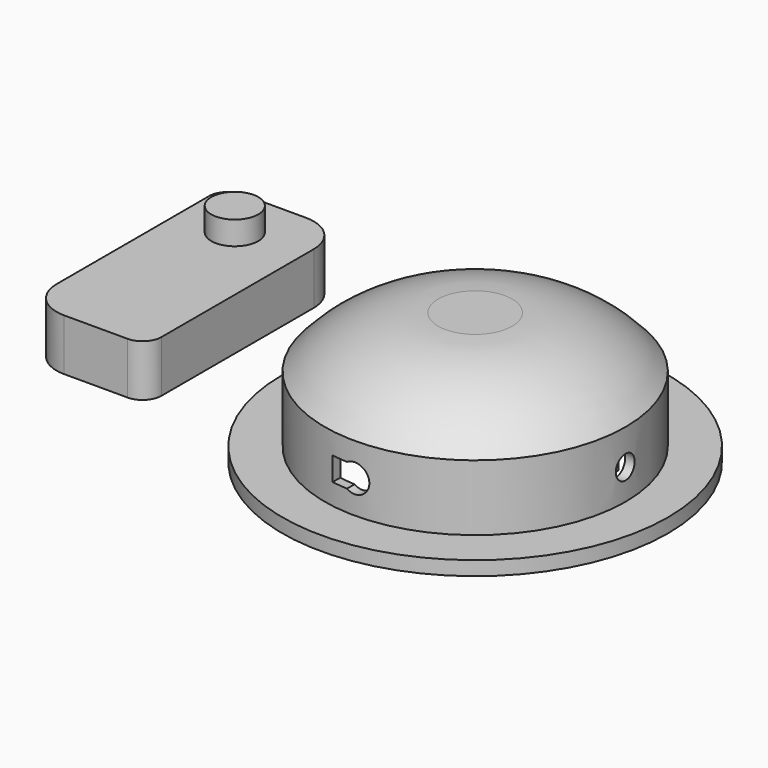
from build123d import *

# Parameters (mm, degrees)
F0_R      = 41
F1_DEPTH  = 3
F2_R      = 32
F3_DEPTH  = 14
F4_R      = 32
F5_DEPTH  = 11
F9_DEPTH  = 120.3
F11_R     = 2.5
F12_DEPTH = 58.4
F13_R     = 40.25
F13_R_2   = 39.25
F14_DEPTH = 1
F15_R     = 39.25
F15_R_2   = 38.75
F16_DEPTH = 0.5
F17_R     = 30
F18_DEPTH = 15
F20_DEPTH = 4.5
F22_DEPTH = 11
F24_DEPTH = 15
F26_DEPTH = 5
F28_DEPTH = 11
F29_R     = 5
F30_DEPTH = 5


# Not quite as in the source:
# - a fillet or chamfer that OpenCascade refuses, or shapes differently, is made with other operations: its cross-section is extruded or revolved along the edge and cut away or added


with BuildPart() as f1:
    # F0 (on Top) → F1 (new body)
    with BuildSketch(Plane.XY):
        Circle(F0_R)
    extrude(amount=F1_DEPTH)

    # F13 (on face) → F14 (cut)
    with BuildSketch(Plane(origin=(0, 0, 0), x_dir=(1, 0, 0), z_dir=(0, 0, -1))):
        Circle(F13_R)
        Circle(F13_R_2, mode=Mode.SUBTRACT)
    extrude(amount=-F14_DEPTH, mode=Mode.SUBTRACT)

    # F15 (on face) → F16 (join)
    with BuildSketch(Plane(origin=(0, 0, 0), x_dir=(1, 0, 0), z_dir=(0, 0, -1))):
        Circle(F15_R)
        Circle(F15_R_2, mode=Mode.SUBTRACT)
    extrude(amount=F16_DEPTH)


with BuildPart() as f3:
    # F2 (on face) → F3 (new body)
    with BuildSketch(Plane.XY.offset(3)):
        Circle(F2_R)
    extrude(amount=F3_DEPTH)

    # F8 (on offset) → F9 (cut)
    with BuildSketch(Plane.XZ.offset(55.4)):
        with BuildLine():
            ThreePointArc((-1.6706518419, 7.5), (1.4062977188, 7.3566179631), (2.9876605533, 10))
            ThreePointArc((2.9876605533, 10), (1.4062977188, 12.6433820369), (-1.6706518419, 12.5))
            ThreePointArc((-1.6706518419, 12.5), (-3.0123394467, 10), (-1.6706518419, 7.5))
        make_face()
        with BuildLine():
            ThreePointArc((-1.6706518419, 7.5), (-3.0123394467, 10), (-1.6706518419, 12.5))
            Line((-1.6706518419, 12.5), (-5.0123394467, 12.5))
            Line((-5.0123394467, 12.5), (-5.0123394467, 10))
            Line((-5.0123394467, 10), (-5.0123394467, 7.5))
            Line((-5.0123394467, 7.5), (-1.6706518419, 7.5))
        make_face()
    extrude(amount=-F9_DEPTH, mode=Mode.SUBTRACT)

    # F11 (on offset) → F12 (cut)
    with BuildSketch(Plane.YZ.offset(56.8)):
        with Locations((0, 9.5)):
            Circle(F11_R)
    extrude(amount=-F12_DEPTH, mode=Mode.SUBTRACT)


with BuildPart() as f5:
    # F4 (on face) → F5 (new body)
    with BuildSketch(Plane.XY.offset(17)):
        Circle(F4_R)
    extrude(amount=F5_DEPTH)

    # F6: fillet of radius 32 on 1 edges, made by hand

    # F6_s1 → F6_t2 (revolve, cut)
    with BuildSketch(Plane.XZ):
        with BuildLine():
            ThreePointArc((32, 17), (21.1211062261, 25.1204395571), (7.8546070647, 28))
            Line((7.8546070647, 28), (32, 28))
            Line((32, 28), (32, 17))
        make_face()
    revolve(axis=Axis((0, 0, 28), (0, 0, 1)), mode=Mode.SUBTRACT)


with BuildPart() as f18_tool:
    # F17 (on face) → F18 (new body)
    with BuildSketch(Plane(origin=(0, 0, 0), x_dir=(1, 0, 0), z_dir=(0, 0, -1))):
        Circle(F17_R)
    extrude(amount=-F18_DEPTH)


with BuildPart() as f1_1:
    add(f1.part)

    # F18: cut by f18_tool
    add(f18_tool.part, mode=Mode.SUBTRACT)

    # F19 (on face) → F20 (join)
    with BuildSketch(Plane(origin=(0, 0, 0), x_dir=(1, 0, 0), z_dir=(0, 0, -1))):
        Polygon((32, 5), (32, 0), (32, -5), (33, -5), (33, 5), align=None)
    extrude(amount=F20_DEPTH)

    # F25 (on face) → F26 (join)
    with BuildSketch(Plane(origin=(0, 0, 0), x_dir=(1, 0, 0), z_dir=(0, 0, -1))):
        with BuildLine():
            Line((5, 30.5941170816), (5, 31.6069612586))
            ThreePointArc((5, 31.6069612586), (0, 32), (-5, 31.6069612586))
            Line((-5, 31.6069612586), (-5, 30.5941170816))
            ThreePointArc((-5, 30.5941170816), (0, 31), (5, 30.5941170816))
        make_face()
        with BuildLine():
            ThreePointArc((-5, -31.6069612586), (0, -32), (5, -31.6069612586))
            Line((5, -31.6069612586), (5, -30.5941170816))
            ThreePointArc((5, -30.5941170816), (0, -31), (-5, -30.5941170816))
            Line((-5, -30.5941170816), (-5, -31.6069612586))
        make_face()
        with BuildLine():
            ThreePointArc((-31.8590646441, -3), (-31.5207631121, -5.5173809756), (-30.9838667697, -8))
            Line((-30.9838667697, -8), (-29.9499582637, -8))
            ThreePointArc((-29.9499582637, -8), (-30.504843096, -5.5185639156), (-30.8544972411, -3))
            Line((-30.8544972411, -3), (-31.8590646441, -3))
        make_face()
        with BuildLine():
            Line((-29.9499582637, 8), (-30.9838667697, 8))
            ThreePointArc((-30.9838667697, 8), (-31.7449502805, 4.0321373594), (-32, 0))
            Line((-32, 0), (-31, 0))
            ThreePointArc((-31, 0), (-30.7363685735, 4.0343087279), (-29.9499582637, 8))
        make_face()
        with BuildLine():
            Line((-31, 0), (-32, 0))
            ThreePointArc((-32, 0), (-31.9960925573, -0.5000610612), (-31.9843711834, -1))
            Line((-31.9843711834, -1), (-30.9838667697, -1))
            ThreePointArc((-30.9838667697, -1), (-30.99596643, -0.500065066), (-31, 0))
        make_face()
    extrude(amount=F26_DEPTH)


with BuildPart() as f3_1:
    add(f3.part)

    # F18: cut by f18_tool
    add(f18_tool.part, mode=Mode.SUBTRACT)

    # F21 (on face) → F22 (join)
    with BuildSketch(Plane(origin=(0, 0, 15), x_dir=(1, 0, 0), z_dir=(0, 0, -1))):
        with BuildLine():
            ThreePointArc((25.25, 6.125), (23.1161165235, 7.0088834765), (24, 4.875))
            ThreePointArc((24, 4.875), (24.8838834765, 5.2411165235), (25.25, 6.125))
        make_face()
        with BuildLine():
            ThreePointArc((24.75, 6.125), (24.5303300859, 5.5946699141), (24, 5.375))
            ThreePointArc((24, 5.375), (23.4696699141, 6.6553300859), (24.75, 6.125))
        make_face(mode=Mode.SUBTRACT)
        with BuildLine():
            ThreePointArc((25.25, -6.125), (24.8838834765, -5.2411165235), (24, -4.875))
            ThreePointArc((24, -4.875), (23.1161165235, -7.0088834765), (25.25, -6.125))
        make_face()
        with BuildLine():
            ThreePointArc((24.75, -6.125), (23.4696699141, -6.6553300859), (24, -5.375))
            ThreePointArc((24, -5.375), (24.5303300859, -5.5946699141), (24.75, -6.125))
        make_face(mode=Mode.SUBTRACT)
    extrude(amount=F22_DEPTH)


with BuildPart() as f24:
    # F23 (on face) → F24 (new body, through all)
    with BuildSketch(Plane(origin=(0, 0, 0), x_dir=(1, 0, 0), z_dir=(0, 0, -1))):
        with BuildLine():
            Line((19.5, 20.25), (18.75, 20.25))
            ThreePointArc((18.75, 20.25), (19.1893398282, 19.1893398282), (20.25, 18.75))
            Line((20.25, 18.75), (20.25, 19.5))
            ThreePointArc((20.25, 19.5), (19.7196699141, 19.7196699141), (19.5, 20.25))
        make_face()
        with BuildLine():
            ThreePointArc((21.6628630048, 20.7538036619), (21.2132034356, 21.2132034356), (20.7538036619, 21.6628630048))
            ThreePointArc((20.7538036619, 21.6628630048), (19.3856231993, 21.475908947), (18.75, 20.25))
            Line((18.75, 20.25), (19.5, 20.25))
            ThreePointArc((19.5, 20.25), (20.25, 21), (21, 20.25))
            ThreePointArc((21, 20.25), (20.7803300859, 19.7196699141), (20.25, 19.5))
            Line((20.25, 19.5), (20.25, 18.75))
            ThreePointArc((20.25, 18.75), (21.3106601718, 19.1893398282), (21.75, 20.25))
            ThreePointArc((21.75, 20.25), (21.7280552268, 20.5056418323), (21.6628630048, 20.7538036619))
        make_face()
    extrude(amount=-F24_DEPTH)


with BuildPart() as f24b:
    # F23 (on face) → F24, piece 2 (new body, through all)
    with BuildSketch(Plane(origin=(0, 0, 0), x_dir=(1, 0, 0), z_dir=(0, 0, -1))):
        with BuildLine():
            Line((19.5, -20.25), (18.75, -20.25))
            ThreePointArc((18.75, -20.25), (19.3856231993, -21.475908947), (20.7538036619, -21.6628630048))
            ThreePointArc((20.7538036619, -21.6628630048), (21.2132034356, -21.2132034356), (21.6628630048, -20.7538036619))
            ThreePointArc((21.6628630048, -20.7538036619), (21.7280552268, -20.5056418323), (21.75, -20.25))
            ThreePointArc((21.75, -20.25), (21.3106601718, -19.1893398282), (20.25, -18.75))
            Line((20.25, -18.75), (20.25, -19.5))
            ThreePointArc((20.25, -19.5), (20.7803300859, -19.7196699141), (21, -20.25))
            ThreePointArc((21, -20.25), (20.25, -21), (19.5, -20.25))
        make_face()
        with BuildLine():
            ThreePointArc((20.25, -18.75), (19.1893398282, -19.1893398282), (18.75, -20.25))
            Line((18.75, -20.25), (19.5, -20.25))
            ThreePointArc((19.5, -20.25), (19.7196699141, -19.7196699141), (20.25, -19.5))
            Line((20.25, -19.5), (20.25, -18.75))
        make_face()
    extrude(amount=-F24_DEPTH)


with BuildPart() as f24c:
    # F23 (on face) → F24, piece 3 (new body, through all)
    with BuildSketch(Plane(origin=(0, 0, 0), x_dir=(1, 0, 0), z_dir=(0, 0, -1))):
        with BuildLine():
            ThreePointArc((-18.75, -20.25), (-19.1893398282, -19.1893398282), (-20.25, -18.75))
            Line((-20.25, -18.75), (-20.25, -19.5))
            ThreePointArc((-20.25, -19.5), (-19.7196699141, -19.7196699141), (-19.5, -20.25))
            Line((-19.5, -20.25), (-18.75, -20.25))
        make_face()
        with BuildLine():
            Line((-20.25, -19.5), (-20.25, -18.75))
            ThreePointArc((-20.25, -18.75), (-21.475908947, -19.3856231993), (-21.6628630048, -20.7538036619))
            ThreePointArc((-21.6628630048, -20.7538036619), (-21.2132034356, -21.2132034356), (-20.7538036619, -21.6628630048))
            ThreePointArc((-20.7538036619, -21.6628630048), (-19.3856231993, -21.475908947), (-18.75, -20.25))
            Line((-18.75, -20.25), (-19.5, -20.25))
            ThreePointArc((-19.5, -20.25), (-20.7803300859, -20.7803300859), (-20.25, -19.5))
        make_face()
    extrude(amount=-F24_DEPTH)


with BuildPart() as f24d:
    # F23 (on face) → F24, piece 4 (new body, through all)
    with BuildSketch(Plane(origin=(0, 0, 0), x_dir=(1, 0, 0), z_dir=(0, 0, -1))):
        with BuildLine():
            Line((-20.25, 19.5), (-20.25, 18.75))
            ThreePointArc((-20.25, 18.75), (-19.1893398282, 19.1893398282), (-18.75, 20.25))
            Line((-18.75, 20.25), (-19.5, 20.25))
            ThreePointArc((-19.5, 20.25), (-19.7196699141, 19.7196699141), (-20.25, 19.5))
        make_face()
        with BuildLine():
            ThreePointArc((-21.6628630048, 20.7538036619), (-21.475908947, 19.3856231993), (-20.25, 18.75))
            Line((-20.25, 18.75), (-20.25, 19.5))
            ThreePointArc((-20.25, 19.5), (-20.7803300859, 20.7803300859), (-19.5, 20.25))
            Line((-19.5, 20.25), (-18.75, 20.25))
            ThreePointArc((-18.75, 20.25), (-19.3856231993, 21.475908947), (-20.7538036619, 21.6628630048))
            ThreePointArc((-20.7538036619, 21.6628630048), (-21.2132034356, 21.2132034356), (-21.6628630048, 20.7538036619))
        make_face()
    extrude(amount=-F24_DEPTH)


with BuildPart() as f28:
    # F27 (on Top) → F28 (new body)
    with BuildSketch(Plane.XY):
        with BuildLine():
            ThreePointArc((-55.5924693942, 26.5955824107), (-57.9356151447, 32.2524366602), (-63.5924693942, 34.5955824107))
            Line((-63.5924693942, 34.5955824107), (-77.0924693942, 34.5955824107))
            ThreePointArc((-77.0924693942, 34.5955824107), (-79.920896519, 33.4240095354), (-81.0924693942, 30.5955824107))
            Line((-81.0924693942, 30.5955824107), (-81.0924693942, -9.9044175893))
            ThreePointArc((-81.0924693942, -9.9044175893), (-78.7493236437, -15.5612718388), (-73.0924693942, -17.9044175893))
            Line((-73.0924693942, -17.9044175893), (-59.5924693942, -17.9044175893))
            ThreePointArc((-59.5924693942, -17.9044175893), (-56.7640422695, -16.7328447141), (-55.5924693942, -13.9044175893))
            Line((-55.5924693942, -13.9044175893), (-55.5924693942, 26.5955824107))
        make_face()
    extrude(amount=F28_DEPTH)

    # F29 (on face) → F30 (join)
    with BuildSketch(Plane.XY.offset(11)):
        with Locations((-69.5924693942, 23.0955824107)):
            Circle(F29_R)
    extrude(amount=F30_DEPTH)


solid = Compound([f5.part, f1_1.part, f3_1.part, f24.part, f24b.part, f24c.part, f24d.part, f28.part])
